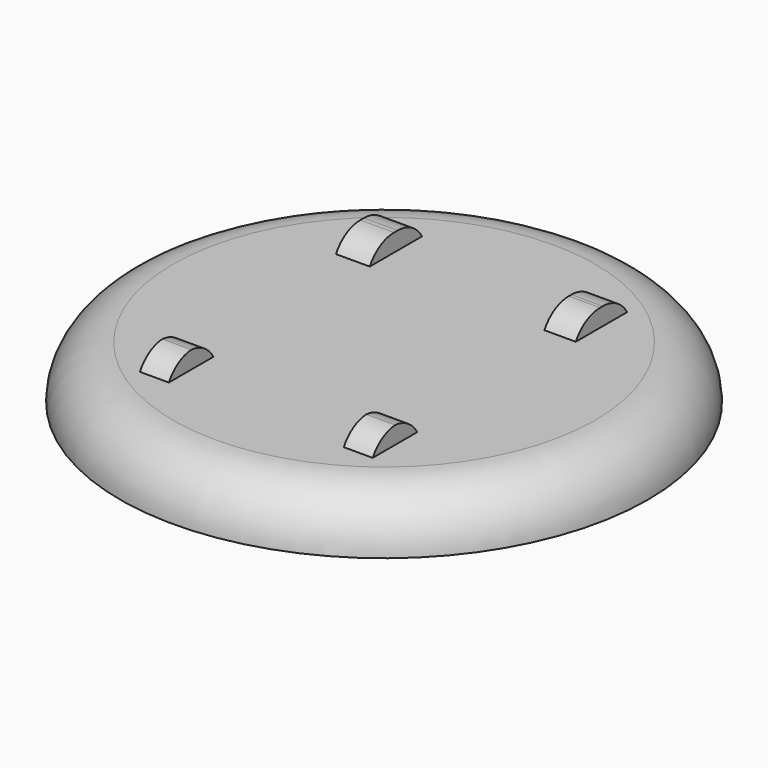
from build123d import *

# Parameters (mm, degrees)
F0_R        = 38.1
F0_W        = 4.1789766401
F0_H        = 8.0406331347
F0_W_2      = 4.8754736781
F0_H_2      = 9.433625348
F0_W_3      = 4.5272270218
F0_H_3      = 9.2595015542
F1_DEPTH    = 7.62
F2_R        = 7.61999
F3_DEPTH    = 10.16
F4_T1_DEPTH = 26.1760218962
F4_T3_DEPTH = 26.1760218962
F4_T5_DEPTH = 26.5242722779
F4_T7_DEPTH = 26.8725189342


# Not quite as in the source:
# - a fillet or chamfer that OpenCascade refuses, or shapes differently, is made with other operations: its cross-section is extruded or revolved along the edge and cut away or added
# - a fillet or chamfer is up to 0.001 mm smaller than in the source, because OpenCascade refuses the exact size


with BuildPart() as f1:
    # F0 (on Top) → F1 (new body)
    with BuildSketch(Plane.XY):
        Circle(F0_R)
        with Locations((-14.8876057938, -18.8208604642)):
            Rectangle(F0_W, F0_H, mode=Mode.SUBTRACT)
        with Locations((14.5393563434, -18.8208604642)):
            Rectangle(F0_W, F0_H, mode=Mode.SUBTRACT)
        with Locations((-15.2358543128, 18.1243643575)):
            Rectangle(F0_W_2, F0_H_2, mode=Mode.SUBTRACT)
        with Locations((14.5393586718, 18.2114262544)):
            Rectangle(F0_W_3, F0_H_3, mode=Mode.SUBTRACT)
    extrude(amount=F1_DEPTH)

    # F2 (radius 7.62 in the source; OpenCascade refuses exactly that, so slightly less here)
    f2_edges = [f1.edges().sort_by_distance(p)[0] for p in [
        (-38.1, 0, 7.62),
    ]]
    fillet(f2_edges, radius=F2_R)

    # F0 (on Top) → F3 (join)
    with BuildSketch(Plane.XY):
        with Locations((-15.2358543128, 18.1243643575)):
            Rectangle(F0_W_2, F0_H_2)
        with Locations((14.5393586718, 18.2114262544)):
            Rectangle(F0_W_3, F0_H_3)
        with Locations((14.5393563434, -18.8208604642)):
            Rectangle(F0_W, F0_H)
        with Locations((-14.8876057938, -18.8208604642)):
            Rectangle(F0_W, F0_H)
    extrude(amount=F3_DEPTH)

    # F4: fillet of radius 5.08 on 8 edges, made by hand

    # F4_s2 → F4_t1 (cut)
    with BuildSketch(Plane.YZ.offset(-27.9756167419)):
        with BuildLine():
            ThreePointArc((-22.8411770315, 7.62), (-20.9817679803, 9.4794090512), (-18.4417679803, 10.16))
            Line((-18.4417679803, 10.16), (-22.8411770315, 10.16))
            Line((-22.8411770315, 10.16), (-22.8411770315, 7.62))
        make_face()
        with BuildLine():
            ThreePointArc((-14.8005438969, 7.62), (-16.6599529481, 9.4794090512), (-19.1999529481, 10.16))
            Line((-19.1999529481, 10.16), (-14.8005438969, 10.16))
            Line((-14.8005438969, 10.16), (-14.8005438969, 7.62))
        make_face()
    extrude(amount=F4_T1_DEPTH, mode=Mode.SUBTRACT)

    # F4_s4 → F4_t3 (cut)
    with BuildSketch(Plane.YZ.offset(1.4513453953)):
        with BuildLine():
            ThreePointArc((-22.8411770315, 7.62), (-20.9817679803, 9.4794090512), (-18.4417679803, 10.16))
            Line((-18.4417679803, 10.16), (-22.8411770315, 10.16))
            Line((-22.8411770315, 10.16), (-22.8411770315, 7.62))
        make_face()
        with BuildLine():
            ThreePointArc((-14.8005438969, 7.62), (-16.6599529481, 9.4794090512), (-19.1999529481, 10.16))
            Line((-19.1999529481, 10.16), (-14.8005438969, 10.16))
            Line((-14.8005438969, 10.16), (-14.8005438969, 7.62))
        make_face()
    extrude(amount=F4_T3_DEPTH, mode=Mode.SUBTRACT)

    # F4_s6 → F4_t5 (cut)
    with BuildSketch(Plane.YZ.offset(1.2772225328)):
        with BuildLine():
            ThreePointArc((13.5816754773, 7.62), (15.4410845286, 9.4794090512), (17.9810845286, 10.16))
            Line((17.9810845286, 10.16), (13.5816754773, 10.16))
            Line((13.5816754773, 10.16), (13.5816754773, 7.62))
        make_face()
        with BuildLine():
            ThreePointArc((22.8411770315, 7.62), (20.9817679803, 9.4794090512), (18.4417679803, 10.16))
            Line((18.4417679803, 10.16), (22.8411770315, 10.16))
            Line((22.8411770315, 10.16), (22.8411770315, 7.62))
        make_face()
    extrude(amount=F4_T5_DEPTH, mode=Mode.SUBTRACT)

    # F4_s8 → F4_t7 (cut)
    with BuildSketch(Plane.YZ.offset(-28.6721137799)):
        with BuildLine():
            ThreePointArc((13.4075516835, 7.62), (15.2669607347, 9.4794090512), (17.8069607347, 10.16))
            Line((17.8069607347, 10.16), (13.4075516835, 10.16))
            Line((13.4075516835, 10.16), (13.4075516835, 7.62))
        make_face()
        with BuildLine():
            ThreePointArc((22.8411770315, 7.62), (20.9817679803, 9.4794090512), (18.4417679803, 10.16))
            Line((18.4417679803, 10.16), (22.8411770315, 10.16))
            Line((22.8411770315, 10.16), (22.8411770315, 7.62))
        make_face()
    extrude(amount=F4_T7_DEPTH, mode=Mode.SUBTRACT)


solid = f1.part
